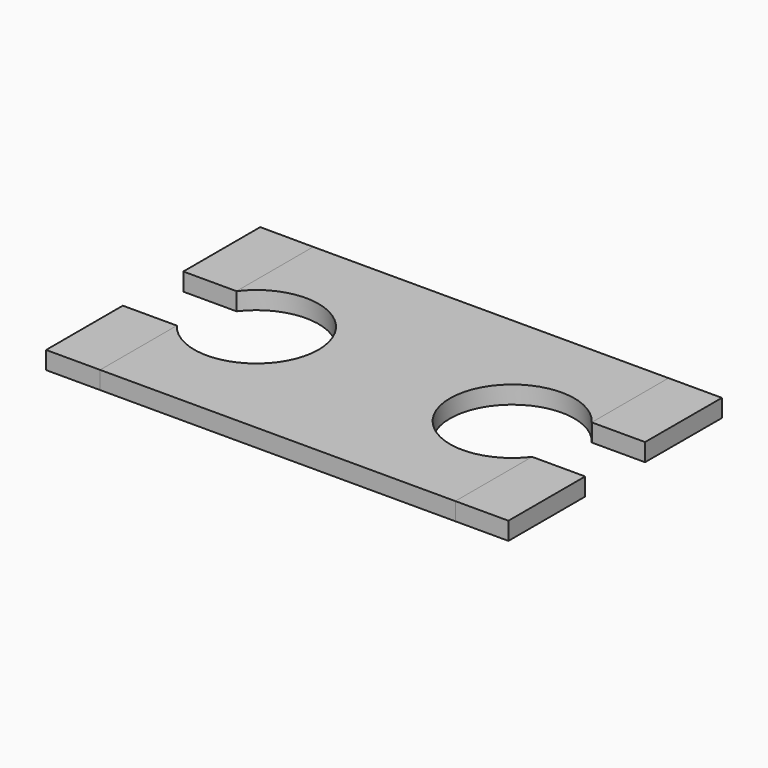
from build123d import *

# Parameters (mm, degrees)
F0_W      = 5.08
F0_H      = 3.81
F1_DEPTH  = 0.254
F3_D      = 1.778
F3_DEPTH  = 25.4
F3_TIP    = 0.5341650903
F5_D      = 1.778
F5_DEPTH  = 25.4
F5_TIP    = 0.5341650903
F7_DEPTH  = 0.254
F9_DEPTH  = 0.254
F10_W     = 0.7592265029
F10_H     = 1.3716
F11_DEPTH = 0.254
F12_W     = 0.7725130153
F12_H     = 1.3716
F13_DEPTH = 0.254


# Not quite as in the source:
# - a feature names something its author has since deleted; it is built from what else it names


with BuildPart() as f1:
    # F0 (on Top) → F1 (new body)
    with BuildSketch(Plane.XY):
        with Locations((-2.54, 1.905)):
            Rectangle(F0_W, F0_H)
    extrude(amount=F1_DEPTH)

    # F3
    with Locations(Plane.XY.offset(0.254)):
        with Locations((-4.3688, 1.905)):
            Hole(F3_D / 2, depth=F3_DEPTH)
            with Locations((0, 0, -(F3_DEPTH + F3_TIP / 2))):  # 118° drill point
                Cone(0, F3_D / 2, F3_TIP, mode=Mode.SUBTRACT)

    # F5
    with Locations(Plane.XY.offset(0.254)):
        with Locations((-0.7112, 1.905)):
            Hole(F5_D / 2, depth=F5_DEPTH)
            with Locations((0, 0, -(F5_DEPTH + F5_TIP / 2))):  # 118° drill point
                Cone(0, F5_D / 2, F5_TIP, mode=Mode.SUBTRACT)


with BuildPart() as f7:
    # F6 (on face) → F7 (new body)
    with BuildSketch(Plane.XY.offset(0.254)):
        Polygon((0.7640526164, 3.81), (0, 3.81), (0, 2.4384), (0.762, 2.4384), align=None)
    extrude(amount=-F7_DEPTH)


with BuildPart() as f9:
    # F8 (on face) → F9 (new body)
    with BuildSketch(Plane.XY.offset(0.254)):
        Polygon((-5.8408910409, 2.4384), (-5.08, 2.4384), (-5.08, 3.81), (-5.8408910409, 3.8134478964), align=None)
    extrude(amount=-F9_DEPTH)


with BuildPart() as f11:
    # F10 (on face) → F11 (new body)
    with BuildSketch(Plane.XY.offset(0.254)):
        with Locations((0.3796132514, 0.6858)):
            Rectangle(F10_W, F10_H)
    extrude(amount=-F11_DEPTH)


with BuildPart() as f13:
    # F12 (on face) → F13 (new body)
    with BuildSketch(Plane.XY.offset(0.254)):
        with Locations((-5.4662565076, 0.6858)):
            Rectangle(F12_W, F12_H)
    extrude(amount=-F13_DEPTH)


solid = Compound([f1.part, f7.part, f9.part, f11.part, f13.part])
